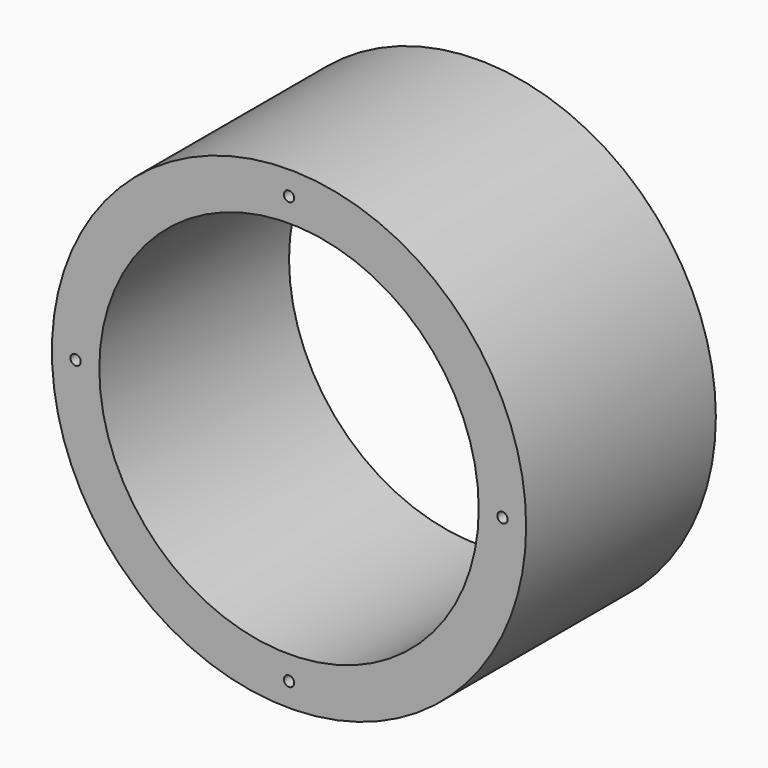
from build123d import *

# Parameters (mm, degrees)
F0_R            = 127
F0_R_2          = 101.6
F1_DEPTH        = 127
F3_D            = 5.5
F3_CBORE_D      = 9.75
F3_CBORE_DEPTH  = 5
F3_COPIES_COUNT = 4


# Not quite as in the source:
# - a pattern or mirror of a feature is missing from the dataset's text; its kind, count and spacing are read off the source's solid


with BuildPart() as f1:
    # F0 (on Front) → F1 (new body)
    with BuildSketch(Plane.XZ):
        Circle(F0_R)
        Circle(F0_R_2, mode=Mode.SUBTRACT)
    extrude(amount=F1_DEPTH)

    # F3 (through all)
    with Locations(Plane(origin=(0, 0, 0), x_dir=(-1, 0, 0), z_dir=(0, 1, 0))):
        with Locations((0, 0), (0, -114.3)):
            f3 = CounterBoreHole(F3_D / 2, F3_CBORE_D / 2, F3_CBORE_DEPTH)

    # F3_copies: F3 ×4 about axis
    f3_copies_axis = Axis((0, 0, 0), (0, 1, 0))
    for i in range(1, F3_COPIES_COUNT):
        add(f3.rotate(f3_copies_axis, i * 360 / F3_COPIES_COUNT), mode=Mode.SUBTRACT)


solid = f1.part
